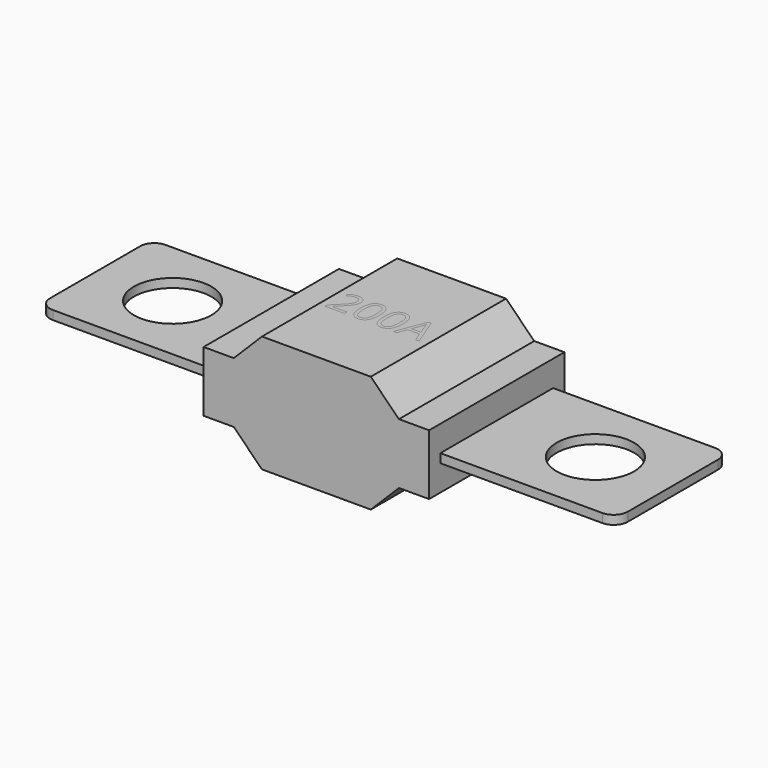
from build123d import *

# Parameters (mm, degrees)
F0_R         = 2.75
F1_DEPTH     = 25
F2_W         = 41.6993834078
F2_H         = 30.2189216949
F3_DEPTH     = 25
F4_TEXT_SIZE = 2.9011786038
F5_DEPTH     = 0.2
F6_DEPTH     = 0.2


# Not quite as in the source:
# - Text() gives the source's letters only with a copy of the font that has no kerning and outlines rounded to 1/6400 em; it was checked with that copy


with BuildPart() as f1:
    # F0 (on Top) → F1 (new body)
    with BuildSketch(Plane.XY):
        with BuildLine():
            Line((8, -5), (19.5, -5))
            ThreePointArc((19.5, -5), (20.2071067812, -4.7071067812), (20.5, -4))
            Line((20.5, -4), (20.5, 4))
            ThreePointArc((20.5, 4), (20.2071067812, 4.7071067812), (19.5, 5))
            Line((19.5, 5), (8, 5))
            Line((8, 5), (8, -5))
        make_face()
        with Locations((15, 0)):
            Circle(F0_R, mode=Mode.SUBTRACT)
        Polygon((8, -6), (8, -5), (8, 5), (8, 6), (-8, 6), (-8, 5), (-8, -5), (-8, -6), align=None)
        with BuildLine():
            Line((-19.5, -5), (-8, -5))
            Line((-8, -5), (-8, 5))
            Line((-8, 5), (-19.5, 5))
            ThreePointArc((-19.5, 5), (-20.2071067812, 4.7071067812), (-20.5, 4))
            Line((-20.5, 4), (-20.5, -4))
            ThreePointArc((-20.5, -4), (-20.2071067812, -4.7071067812), (-19.5, -5))
        make_face()
        with Locations((-15, 0)):
            Circle(F0_R, mode=Mode.SUBTRACT)
    extrude(amount=F1_DEPTH)

    # F2 (on face) → F3 (cut)
    with BuildSketch(Plane.XZ.offset(6)):
        with Locations((0, 12.5)):
            Rectangle(F2_W, F2_H)
        Polygon((20.5, 12.815), (20.5, 12.185), (8, 12.185), (8, 10.35), (5.8605, 10.35), (3.8605, 8.35), (-3.8605, 8.35), (-5.8605, 10.35), (-8, 10.35), (-8, 12.185), (-20.5, 12.185), (-20.5, 12.815), (-8, 12.815), (-8, 14.65), (-5.8605, 14.65), (-3.8605, 16.65), (3.8605, 16.65), (5.8605, 14.65), (8, 14.65), (8, 12.815), align=None, mode=Mode.SUBTRACT)
    extrude(amount=-F3_DEPTH, mode=Mode.SUBTRACT)

    # F4 (on face) → F5 (cut)
    with BuildSketch(Plane.XY.offset(16.65)):
        with Locations((-3.5340312451, -0.9765039904)):
            Text('200A', F4_TEXT_SIZE, font='Open Sans', text_align=(TextAlign.LEFT, TextAlign.BOTTOM))
    extrude(amount=-F5_DEPTH, mode=Mode.SUBTRACT)


with BuildPart() as f6:
    # F6 (new): a face of the model
    f6_faces = [f1.part.faces().sort_by_distance(p)[0] for p in [
        (-2.71150178, -0.951472469, 16.45),
    ]]
    extrude(f6_faces, amount=F6_DEPTH)


with BuildPart() as f6b:
    # F6#2 (new): a face of the model
    f6_2_faces = [f1.part.faces().sort_by_distance(p)[0] for p in [
        (-1.7054221263, 0.0603622053, 16.45),
    ]]
    extrude(f6_2_faces, amount=F6_DEPTH)


with BuildPart() as f6c:
    # F6#3 (new): a face of the model
    f6_3_faces = [f1.part.faces().sort_by_distance(p)[0] for p in [
        (-0.0467639214, 0.0603622053, 16.45),
    ]]
    extrude(f6_3_faces, amount=F6_DEPTH)


with BuildPart() as f6d:
    # F6#4 (new): a face of the model
    f6_4_faces = [f1.part.faces().sort_by_distance(p)[0] for p in [
        (2.9253906204, -0.6370591186, 16.45),
    ]]
    extrude(f6_4_faces, amount=F6_DEPTH)


solid = Compound([f1.part, f6.part, f6b.part, f6c.part, f6d.part])
